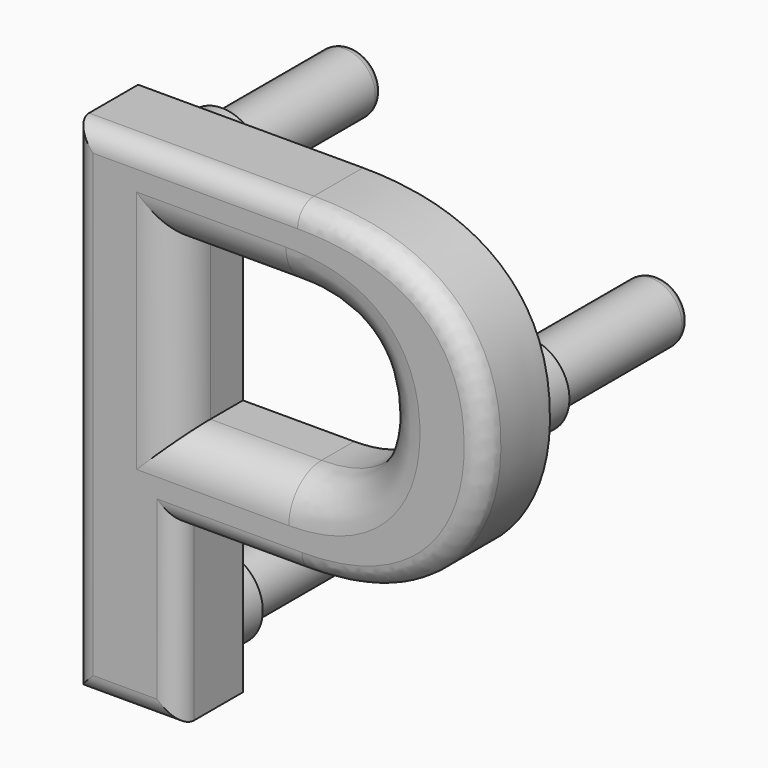
from build123d import *

# Parameters (mm, degrees)
F0_TEXT_SIZE = 35.6030262572
F1_DEPTH     = 4
F2_R         = 2
F3_R         = 1
F4_R         = 1.5
F5_DEPTH     = 10
F6_R         = 2
F7_DEPTH     = 2
F8_R         = 0.5


# Not quite as in the source:
# - a feature names something its author has since deleted; it is built from what else it names
# - Text() gives the source's letters only with a copy of the font that has no kerning and outlines rounded to 1/6400 em; it was checked with that copy


with BuildPart() as f1:
    # F0 (on Front) → F1 (new body)
    with BuildSketch(Plane.XZ):
        with Locations((-7.0323857276, -16.9004096178)):
            Text('P', F0_TEXT_SIZE, font='Arimo', font_style=FontStyle.BOLD, text_align=(TextAlign.LEFT, TextAlign.BOTTOM))
    extrude(amount=F1_DEPTH)

    # F2
    f2_edges = [f1.edges().sort_by_distance(p)[0] for p in [
        (3.197921, -4, -4.333654),
        (0.477628, -4, -0.35891),
    ]]
    fillet(f2_edges, radius=F2_R)

    # F3
    f3_edges = [f1.edges().sort_by_distance(p)[0] for p in [
        (0.477628, -4, -12.589106),
        (-2.086903, -4, -16.90041),
        (-4.651433, -4, -4.653525),
        (14.961607, -4, 2.98109),
    ]]
    fillet(f3_edges, radius=F3_R)

    # F4 (on face) → F5 (join)
    with BuildSketch(Plane(origin=(0, 0, 0), x_dir=(-1, 0, 0), z_dir=(0, 1, 0))):
        with Locations((2.1514333466, 4.5933598526)):
            Circle(F4_R)
        with Locations((-12.8485666534, -0.4066401474)):
            Circle(F4_R)
        with Locations((2.1514333466, -14.4066401474)):
            Circle(F4_R)
    extrude(amount=F5_DEPTH)

    # F6 (on face) → F7 (join)
    with BuildSketch(Plane(origin=(0, 0, 0), x_dir=(-1, 0, 0), z_dir=(0, 1, 0))):
        with Locations((2.1514333466, 4.5933598526)):
            Circle(F6_R)
        with Locations((-12.8485666534, -0.4066401474)):
            Circle(F6_R)
        with Locations((2.1514333466, -14.4066401474)):
            Circle(F6_R)
    extrude(amount=F7_DEPTH)

    # F8
    f8_edges = [f1.edges().sort_by_distance(p)[0] for p in [
        (-0.651433, 10, 4.59336),
        (-0.651433, 10, -14.40664),
        (14.348567, 10, -0.40664),
    ]]
    fillet(f8_edges, radius=F8_R)


solid = f1.part
